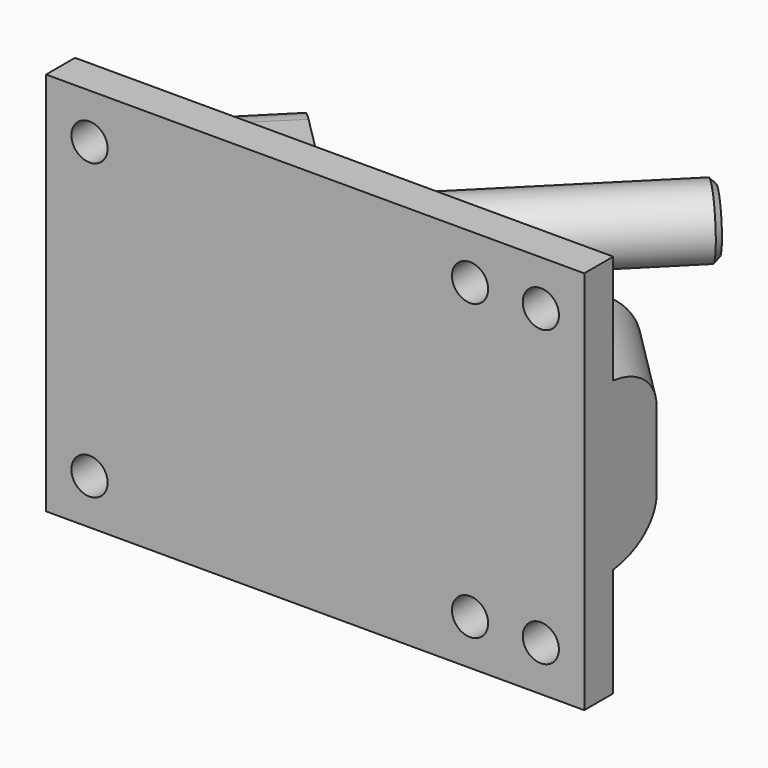
from build123d import *

# Parameters (mm, degrees)
F1_DEPTH = 27.0002
F2_R     = 9.906
F3_W     = 75.565
F3_H     = 31.9504877579
F4_DEPTH = 15.24
F5_R     = 2.54
F6_DEPTH = 5.081
F8_R     = 6.35
F14_SIZE = 0.762


with BuildPart() as f1:
    # F0 (on Top) → F1 (new body)
    with BuildSketch(Plane.XY):
        Polygon((64.7048964237, 23.5601035763), (42.2542561211, 1.1094632736), (6.3332316368, 37.0304877579), (0, 30.6972561211), (0, 0), (75.565, 0), (75.565, 12.7), align=None)
    extrude(amount=-F1_DEPTH)

    # F2
    f2_edges = [f1.edges().sort_by_distance(p)[0] for p in [
        (42.254256, 1.109463, -13.5001),
    ]]
    fillet(f2_edges, radius=F2_R)

    # F3 (on Top) → F4 (cut)
    with BuildSketch(Plane.XY):
        with Locations((37.7825, 21.0552438789)):
            Rectangle(F3_W, F3_H)
    extrude(amount=-F4_DEPTH, mode=Mode.SUBTRACT)

    # F5 (on face) → F6 (cut, through all)
    with BuildSketch(Plane(origin=(0, 5.08, 0), x_dir=(-1, 0, 0), z_dir=(0, 1, 0))):
        with Locations((-69.469, -6.35)):
            Circle(F5_R)
        with Locations((-59.5265105367, -6.35)):
            Circle(F5_R)
        with Locations((-6.096, -6.35)):
            Circle(F5_R)
    extrude(amount=-F6_DEPTH, mode=Mode.SUBTRACT)

    # F7: F1 across face


with BuildPart() as f1_1:
    add(f1.part)
    add(f1.part.mirror(Plane(origin=(31.4297936493, 11.6265989231, -27.0002), x_dir=(1, 0, 0), z_dir=(0, 0, -1))))

    # F8
    f8_edges = [f1_1.edges().sort_by_distance(p)[0] for p in [
        (70.134948, 18.130052, -38.7604),
        (70.134948, 18.130052, -15.24),
        (3.166616, 33.863872, -38.7604),
        (3.166616, 33.863872, -15.24),
    ]]
    fillet(f8_edges, radius=F8_R)


with BuildPart() as f1_2:
    # F10: moved
    add(f1_1.part.moved(Location((0, 0, 27.0002))))

    # F9 (on Top) → F11 (revolve, cut)
    with BuildSketch(Plane.XY):
        Polygon((-6.3683719395, 6.3683719395), (15.3134877579, 28.0502316368), (11.9458917125, 31.4178276822), (5.2106996217, 24.6826355914), (2.6782673955, 27.2150678175), (-12.268400211, 12.268400211), align=None)
    revolve(axis=Axis((22.0486798487, 34.7854237276, 0), (0.7071067812, 0.7071067812, 0)), mode=Mode.SUBTRACT)

    # F15 (on Top) → F16 (revolve, cut)
    with BuildSketch(Plane.XY):
        Polygon((64.7048964237, 5.5995913341), (70.0930500964, 10.9877450068), (61.1127939753, 19.9680011278), (55.7246403027, 14.5798474552), align=None)
    revolve(axis=Axis((60.2147683632, 10.0897193947, 0), (-0.7071067812, 0.7071067812, 0)), mode=Mode.SUBTRACT)


with BuildPart() as f13:
    # F12 (on Top) → F13 (revolve)
    with BuildSketch(Plane.XY):
        Polygon((5.2106996217, 24.6826355914), (2.9656355914, 26.9276996217), (1.1695843672, 25.1316483974), (6.7822444428, 19.5189883218), (46.7443841816, 59.4811280605), (43.3767881362, 62.8487241059), (11.9458917125, 31.4178276822), align=None)
    revolve(axis=Axis((26.7633143122, 39.5000581912, 0), (0.7071067812, 0.7071067812, 0)))

    # F14
    f14_edges = [f13.edges().sort_by_distance(p)[0] for p in [
        (50.11198, 56.113532, 0),
    ]]
    chamfer(f14_edges, length=F14_SIZE)


with BuildPart() as f19:
    # F18 (on Top) → F19 (revolve)
    with BuildSketch(Plane.XY):
        with BuildLine():
            Line((62.0108195874, 8.2936681704), (64.7048964237, 5.5995913341))
            Line((64.7048964237, 5.5995913341), (70.0930500964, 10.9877450068))
            Line((70.0930500964, 10.9877450068), (61.1127939753, 19.9680011278))
            Line((61.1127939753, 19.9680011278), (60.2147683632, 19.0699755157))
            Line((60.2147683632, 19.0699755157), (59.3167427511, 18.1719499036))
            Line((59.3167427511, 18.1719499036), (62.0108195874, 15.4778730673))
            ThreePointArc((62.0108195874, 15.4778730673), (63.498717139, 11.8857706189), (62.0108195874, 8.2936681704))
        make_face()
    revolve(axis=Axis((40.0091920908, 30.2952956671, 0), (-0.7071067812, 0.7071067812, 0)))


solid = Compound([f1_2.part, f13.part, f19.part])
